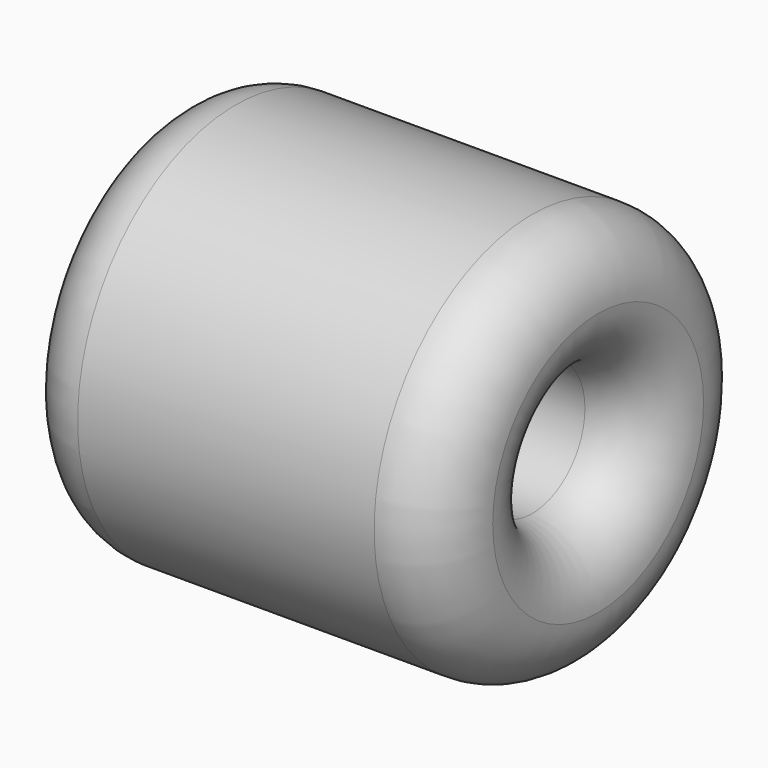
from build123d import *

# Parameters (mm, degrees)
F0_R     = 30
F0_R_2   = 10
F1_DEPTH = 65
F2_R     = 9.99999


# Not quite as in the source:
# - a fillet or chamfer is up to 0.001 mm smaller than in the source, because OpenCascade refuses the exact size


with BuildPart() as f1:
    # F0 (on Right) → F1 (new body)
    with BuildSketch(Plane.YZ):
        Circle(F0_R)
        Circle(F0_R_2, mode=Mode.SUBTRACT)
    extrude(amount=F1_DEPTH)

    # F2 (radius 10 in the source; OpenCascade refuses exactly that, so slightly less here)
    f2_edges = [f1.edges().sort_by_distance(p)[0] for p in [
        (65, -30, 0),
        (65, -10, 0),
        (32.5, 30, 0),
        (0, -30, 0),
        (0, -10, 0),
        (32.5, 10, 0),
    ]]
    fillet(f2_edges, radius=F2_R)


solid = f1.part
